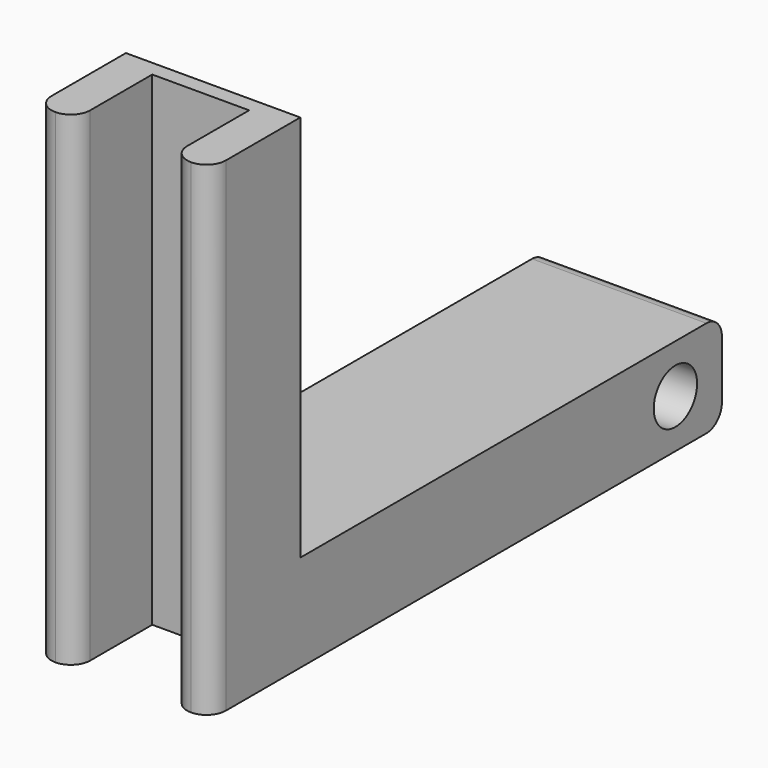
from build123d import *

# Parameters (mm, degrees)
F1_DEPTH = 25
F0_W     = 9
F0_H     = 27.2
F2_DEPTH = 5
F3_R     = 1.4
F4_DEPTH = 12.5
F5_R     = 0.99999


# Not quite as in the source:
# - a fillet or chamfer is up to 0.001 mm smaller than in the source, because OpenCascade refuses the exact size


with BuildPart() as f1:
    # F0 (on Top) → F1 (new body)
    with BuildSketch(Plane.XY):
        Polygon((-4.5, 5.8), (-4.5, 0), (-2.5, 0), (-2.5, 5), (2.5, 5), (2.5, 0), (4.5, 0), (4.5, 5.8), align=None)
    extrude(amount=F1_DEPTH)

    # F0 (on Top) → F2 (join)
    with BuildSketch(Plane.XY):
        with Locations((0, 19.4)):
            Rectangle(F0_W, F0_H)
    extrude(amount=F2_DEPTH)

    # F3 (on Right) → F4 (cut, symmetric)
    with BuildSketch(Plane.YZ):
        with Locations((30, 2.5)):
            Circle(F3_R)
    extrude(amount=F4_DEPTH, both=True, mode=Mode.SUBTRACT)

    # F5 (radius 1 in the source; OpenCascade refuses exactly that, so slightly less here)
    f5_edges = [f1.edges().sort_by_distance(p)[0] for p in [
        (0, 33, 5),
        (0, 33, 0),
        (-2.5, 0, 12.5),
        (2.5, 0, 12.5),
        (-4.5, 0, 12.5),
        (4.5, 0, 12.5),
    ]]
    fillet(f5_edges, radius=F5_R)


solid = f1.part
